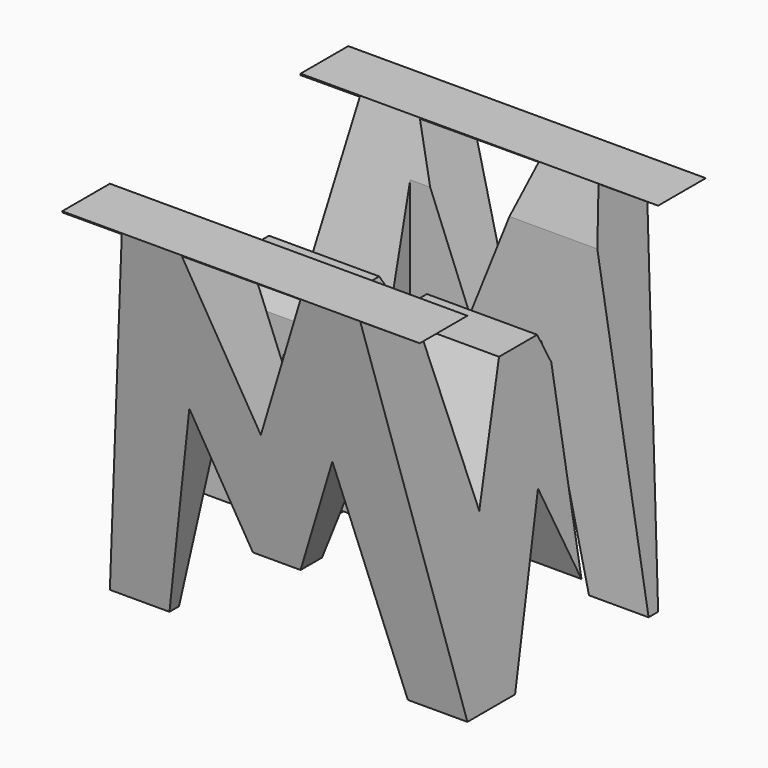
from build123d import *

# Parameters (mm, degrees)
F0_W      = 38.1
F0_H      = 38.1
F1_DEPTH  = 38.1
F6_DEPTH  = 38.1
F9_DEPTH  = 38.1
F10_W     = 25.4
F10_H     = 7.62
F11_DEPTH = 38.1


with BuildPart() as f1:
    # F0 (on Front) → F1 (new body)
    with BuildSketch(Plane.XZ):
        with Locations((19.05, 19.05)):
            Rectangle(F0_W, F0_H)
    extrude(amount=F1_DEPTH)

    # F5 (on offset) → F6 (cut)
    with BuildSketch(Plane.YZ.offset(38.1)):
        Polygon((-6.35, 38.1), (-31.75, 38.1), (-26.67, 16.8241550819), (-21.59, 28.575), (-16.51, 28.575), (-11.43, 16.8241550819), align=None)
        Polygon((-31.75, 0), (-38.1, 38.1), (-38.1, 0), align=None)
        Polygon((-19.05, 15.875), (-25.4, 0), (-22.9262417018, 0), (-19.05, 0), (-12.7, 0), align=None)
        Polygon((0, 0), (0, 38.1), (-6.35, 0), align=None)
    extrude(amount=-F6_DEPTH, mode=Mode.SUBTRACT)

    # F8 (on face) → F9 (cut)
    with BuildSketch(Plane.XZ.offset(38.1)):
        Polygon((0, 37.9714828326), (0, 0), (6.3321403529, 37.9928421172), align=None)
        Polygon((11.43, 22.225), (6.35, 0), (31.75, 0), (26.67, 22.225), (21.59, 9.525), (16.51, 9.525), align=None)
        Polygon((25.382841226, 38.057103065), (12.7342250661, 38.0144373348), (19.05, 22.225), align=None)
        Polygon((31.7535679155, 38.0785925072), (38.1, 0), (38.1, 38.1), align=None)
    extrude(amount=-F9_DEPTH, mode=Mode.SUBTRACT)

    # F10 (on offset) → F11 (cut)
    with BuildSketch(Plane.XY.offset(38.1)):
        with Locations((25.4, -11.43)):
            Rectangle(F10_W, F10_H)
        with Locations((12.7, -26.67)):
            Rectangle(F10_W, F10_H)
    extrude(amount=-F11_DEPTH, mode=Mode.SUBTRACT)


solid = f1.part
